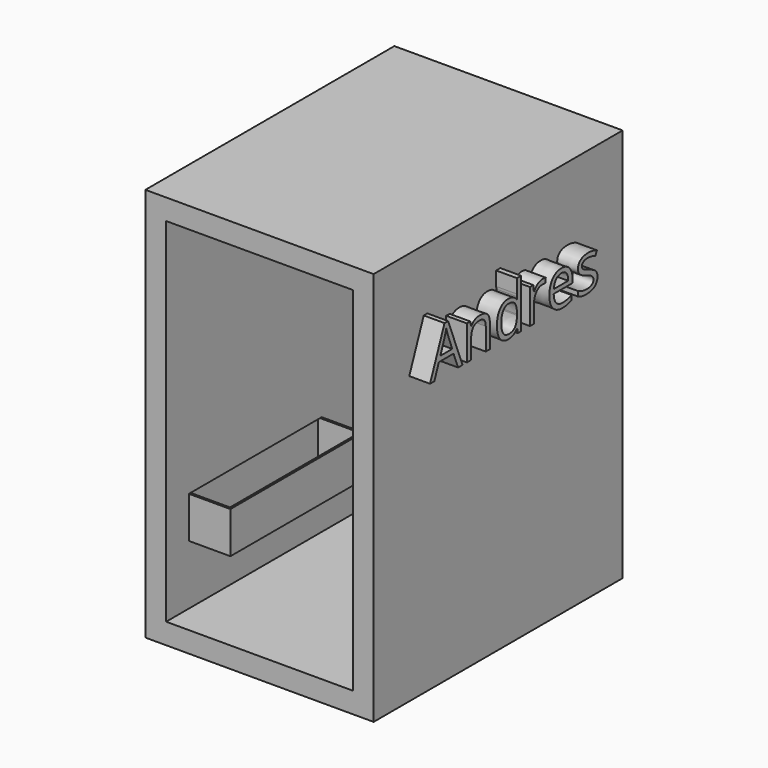
from build123d import *

# Parameters (mm, degrees)
F1_DEPTH      = 381
F2_T          = -25.4
F3_W          = 203.2
F3_H          = 50.8
F4_DEPTH      = 50.8
F5_T          = 2.54
F5_T3_DEPTH   = 360.68
F5_T5_DEPTH   = 233.68
F5_T7_DEPTH   = 436.88
F5_T9_DEPTH   = 55.88
F5_T11_DEPTH  = 208.28
F6_W          = 50.8
F6_H          = 25.4
F7_DEPTH      = 25.4
F8_R          = 6.35
F9_DEPTH      = 25.4
F10_TEXT_SIZE = 78.5984926754
F11_DEPTH     = 25.4
F12_TEXT_SIZE = 64.1105489598
F13_DEPTH     = 25.4
F14_W         = 50.8
F14_H         = 50.8
F15_DEPTH     = 50.8
F16_R         = 20.681616161
F17_DEPTH     = 45.72


# Not quite as in the source:
# - a shell that OpenCascade refuses in one call is made with other operations: the cavity is built on its own and cut out
# - Text() gives the source's letters only with a copy of the font that has no kerning and outlines rounded to 1/6400 em; it was checked with that copy


with BuildPart() as f1:
    # F0 (on Front) → F1 (new body)
    with BuildSketch(Plane.XZ):
        Polygon((-139.7, 0), (0, 0), (139.7, 0), (139.7, 482.6), (-139.7, 482.6), align=None)
    extrude(amount=F1_DEPTH)

    # F2
    f2_openings = [f1.faces().sort_by_distance(p)[0] for p in [
        (0, -381, 241.3),
    ]]
    offset(amount=F2_T, openings=f2_openings)

    # F3 (on face) → F4 (join)
    with BuildSketch(Plane.YZ.offset(-114.3)):
        with Locations((-244.5578786373, 123.6916609764)):
            Rectangle(F3_W, F3_H)
    extrude(amount=F4_DEPTH)

    # F5: shell of thickness 2.54, made by hand


with BuildPart() as f5_core1:
    # F5_t2: copy of F1
    add(f1.part)

    # the walls: a layer under each face that stays
    f5_faces = [f5_core1.faces().sort_by_distance(p)[0] for p in [
        (0, -190.5, 0),
        (-139.7, -190.5, 241.3),
        (-119.7428571429, -381, 34.4714285714),
        (139.7, -190.5, 241.3),
        (0, 0, 241.3),
        (0, -190.5, 482.6),
        (0, -203.2, 457.2),
        (114.3, -203.2, 241.3),
        (0, -203.2, 25.4),
        (-114.3, -203.2, 241.3),
        (0, -25.4, 241.3),
        (-88.9, -346.1578786373, 123.6916609764),
        (-88.9, -244.5578786373, 98.2916609764),
        (-88.9, -142.9578786373, 123.6916609764),
        (-63.5, -244.5578786373, 123.6916609764),
    ]]
    thicken(f5_faces, amount=-F5_T, mode=Mode.SUBTRACT)

    # F5_s4 → F5_t3 (cut)
    with BuildSketch(Plane.XZ.offset(22.86)):
        Polygon((-114.2746, 457.1746), (-114.3, 459.74), (-116.84, 459.74), (-116.84, 457.2), align=None)
        Polygon((114.2746, 457.1746), (114.3, 459.74), (116.84, 459.74), (116.84, 457.2), align=None)
        Polygon((114.2746, 25.4254), (116.84, 25.4), (116.84, 22.86), (114.3, 22.86), align=None)
        Polygon((-114.2746, 25.4254), (-114.3, 22.86), (-116.84, 22.86), (-116.84, 25.4), align=None)
    extrude(amount=F5_T3_DEPTH, mode=Mode.SUBTRACT)

    # F5_s6 → F5_t5 (cut)
    with BuildSketch(Plane.YZ.offset(-116.84)):
        Polygon((-25.4254, 457.1746), (-25.4, 459.74), (-22.86, 459.74), (-22.86, 457.2), align=None)
        Polygon((-25.4254, 25.4254), (-25.4, 22.86), (-22.86, 22.86), (-22.86, 25.4), align=None)
    extrude(amount=F5_T5_DEPTH, mode=Mode.SUBTRACT)

    # F5_s8 → F5_t7 (cut)
    with BuildSketch(Plane.XY.offset(22.86)):
        Polygon((114.2746, -25.4254), (116.84, -25.4), (116.84, -22.86), (114.3, -22.86), align=None)
        Polygon((-114.2746, -25.4254), (-116.84, -25.4), (-116.84, -22.86), (-114.3, -22.86), align=None)
    extrude(amount=F5_T7_DEPTH, mode=Mode.SUBTRACT)

    # F5_s10 → F5_t9 (cut)
    with BuildSketch(Plane.XY.offset(95.7516609764)):
        Polygon((-114.2746, -346.1832786373), (-116.84, -346.1578786373), (-116.84, -343.6178786373), (-114.3, -343.6178786373), align=None)
        Polygon((-114.2746, -142.9324786373), (-116.84, -142.9578786373), (-116.84, -145.4978786373), (-114.3, -145.4978786373), align=None)
    extrude(amount=F5_T9_DEPTH, mode=Mode.SUBTRACT)

    # F5_s12 → F5_t11 (cut)
    with BuildSketch(Plane.XZ.offset(140.4178786373)):
        Polygon((-114.2746, 98.2662609764), (-116.84, 98.2916609764), (-116.84, 100.8316609764), (-114.3, 100.8316609764), align=None)
    extrude(amount=F5_T11_DEPTH, mode=Mode.SUBTRACT)


with BuildPart() as f1_1:
    add(f1.part)

    # what is left inside the walls is the cavity
    f5_cavity = [f5_core1.part.solids().sort_by_distance(p)[0] for p in [
        (-137.1346, -253.153333, 241.3),
    ]]
    add(f5_cavity, mode=Mode.SUBTRACT)

    # F6 (on face) → F7 (join)
    with BuildSketch(Plane(origin=(114.3, 0, 0), x_dir=(0, -1, 0), z_dir=(-1, 0, 0))):
        with Locations((230.5243931055, 155.6519333601)):
            Rectangle(F6_W, F6_H)
    extrude(amount=F7_DEPTH)

    # F8 (on face) → F9 (cut)
    with BuildSketch(Plane.XY.offset(168.3519333601)):
        with Locations((102.9301136732, -230.5243931055)):
            Circle(F8_R)
    extrude(amount=-F9_DEPTH, mode=Mode.SUBTRACT)

    # F10 (on face) → F11 (join)
    with BuildSketch(Plane.YZ.offset(139.7)):
        with Locations((-326.4489471912, 350.5174517632)):
            Text('Andres', F10_TEXT_SIZE, font='Open Sans', text_align=(TextAlign.LEFT, TextAlign.BOTTOM))
    extrude(amount=F11_DEPTH)

    # F12 (on face) → F13 (join)
    with BuildSketch(Plane(origin=(-139.7, 0, 0), x_dir=(0, -1, 0), z_dir=(-1, 0, 0))):
        with Locations((22.6401984692, 366.8102025986)):
            Text('Fernandez', F12_TEXT_SIZE, font='Open Sans', text_align=(TextAlign.LEFT, TextAlign.BOTTOM))
    extrude(amount=F13_DEPTH)

    # F14 (on face) → F15 (join)
    with BuildSketch(Plane.XZ.offset(25.4)):
        with Locations((-11.9700000346, 112.1731527805)):
            Rectangle(F14_W, F14_H)
    extrude(amount=F15_DEPTH)

    # F16 (on face) → F17 (cut)
    with BuildSketch(Plane.XY.offset(137.5731527805)):
        with Locations((-11.3794645295, -49.2739714682)):
            Circle(F16_R)
    extrude(amount=-F17_DEPTH, mode=Mode.SUBTRACT)


solid = f1_1.part
